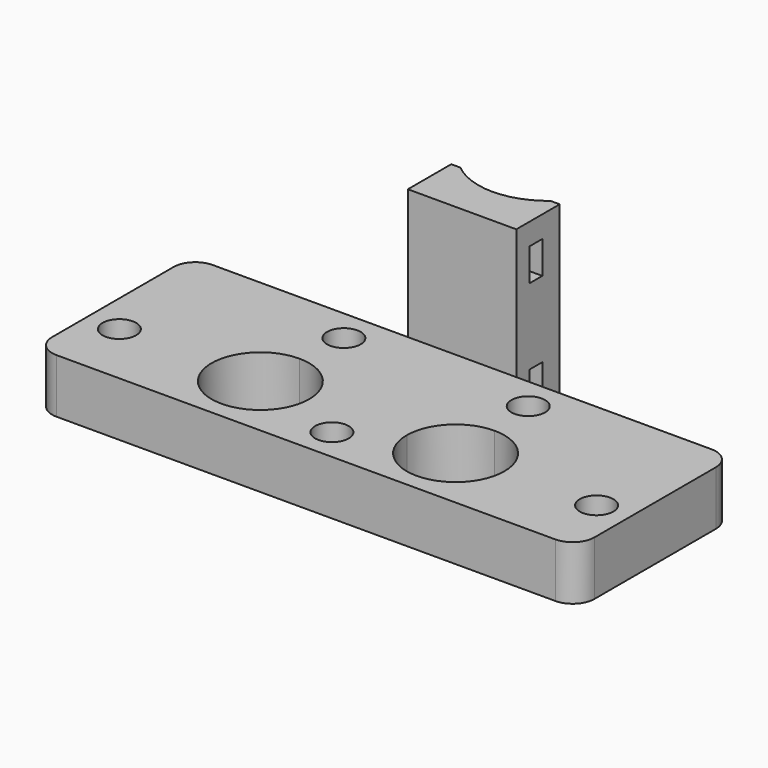
from build123d import *

# Parameters (mm, degrees)
F0_R          = 1.55
F1_DEPTH      = 5
F2_DEPTH      = 4
F3_DEPTH      = 17
F4_W          = 1.5
F4_H          = 3
F5_DEPTH      = 25
F6_W          = 1.52
F6_H          = 2
F7_DEPTH      = 11
F8_F1_R       = 2
F8_F2_R       = 2
F8_F3_R       = 2
F8_F4_R       = 2
F8_2_T1_DEPTH = 14


# Not quite as in the source:
# - a fillet or chamfer that OpenCascade refuses, or shapes differently, is made with other operations: its cross-section is extruded or revolved along the edge and cut away or added
# - a feature names something its author has since deleted; it is built from what else it names


with BuildPart() as f1:
    # F0 (on Top) → F1 (new body)
    with BuildSketch(Plane.XY):
        Polygon((-10, 0), (0, 0), (0, 10.5), (0, 18), (-10, 18), align=None)
        with Locations((-7, 6)):
            Circle(F0_R, mode=Mode.SUBTRACT)
        with BuildLine():
            Line((0, 10.5), (0, 0))
            Line((0, 0), (10.5, 0))
            Line((10.5, 0), (10.5, 6))
            ThreePointArc((10.5, 6), (2.8180194847, 2.8180194847), (6, 10.5))
            Line((6, 10.5), (0, 10.5))
        make_face()
        with BuildLine():
            Line((10.5, 6), (10.5, 0))
            Line((10.5, 0), (19.5, 0))
            Line((19.5, 0), (19.5, 6))
            ThreePointArc((19.5, 6), (20.8180194847, 9.1819805153), (24, 10.5))
            Line((24, 10.5), (6, 10.5))
            ThreePointArc((6, 10.5), (9.1819805153, 9.1819805153), (10.5, 6))
        make_face()
        with Locations((15, 3)):
            Circle(F0_R, mode=Mode.SUBTRACT)
        with BuildLine():
            Line((19.5, 6), (19.5, 0))
            Line((19.5, 0), (30, 0))
            Line((30, 0), (30, 10.5))
            Line((30, 10.5), (24, 10.5))
            ThreePointArc((24, 10.5), (27.1819805153, 9.1819805153), (28.5, 6))
            ThreePointArc((28.5, 6), (24, 1.5), (19.5, 6))
        make_face()
        Polygon((30, 10.5), (30, 0), (40, 0), (40, 18), (30, 18), align=None)
        with Locations((37, 6)):
            Circle(F0_R, mode=Mode.SUBTRACT)
        Polygon((0, 18), (0, 10.5), (6, 10.5), (24, 10.5), (30, 10.5), (30, 18), (20, 18), (10, 18), align=None)
        with Locations((6.5, 15)):
            Circle(F0_R, mode=Mode.SUBTRACT)
        with Locations((23.5, 15)):
            Circle(F0_R, mode=Mode.SUBTRACT)
    extrude(amount=F1_DEPTH)

    # F0 (on Top) → F3 (join)
    with BuildSketch(Plane.XY):
        with BuildLine():
            Line((10, 23), (10, 18))
            Line((10, 18), (20, 18))
            Line((20, 18), (20, 23))
            Line((20, 23), (19.1533119315, 23))
            ThreePointArc((19.1533119315, 23), (15, 21.5), (10.8466880685, 23))
            Line((10.8466880685, 23), (10, 23))
        make_face()
    extrude(amount=F3_DEPTH)

    # F4 (on face) → F5 (cut)
    with BuildSketch(Plane(origin=(10, 0, 0), x_dir=(0, -1, 0), z_dir=(-1, 0, 0))):
        with Locations((-20.25, 3.5)):
            Rectangle(F4_W, F4_H)
        with Locations((-20.25, 13.5)):
            Rectangle(F4_W, F4_H)
    extrude(amount=-F5_DEPTH, mode=Mode.SUBTRACT)

    # F8: fillet of radius 2 on 4 edges, made by hand

    # F8_f1
    f8_f1_edges = [f1.edges().sort_by_distance(p)[0] for p in [
        (40, 0, 2.5),
    ]]
    fillet(f8_f1_edges, radius=F8_F1_R)

    # F8_f2
    f8_f2_edges = [f1.edges().sort_by_distance(p)[0] for p in [
        (40, 18, 2.5),
    ]]
    fillet(f8_f2_edges, radius=F8_F2_R)

    # F8_f3
    f8_f3_edges = [f1.edges().sort_by_distance(p)[0] for p in [
        (-10, 0, 2.5),
    ]]
    fillet(f8_f3_edges, radius=F8_F3_R)

    # F8_f4
    f8_f4_edges = [f1.edges().sort_by_distance(p)[0] for p in [
        (-10, 18, 2.5),
    ]]
    fillet(f8_f4_edges, radius=F8_F4_R)


with BuildPart() as f2:
    # F0 (on Top) → F2 (new body)
    with BuildSketch(Plane.XY):
        Polygon((0, 18), (0, 10.5), (6, 10.5), (24, 10.5), (30, 10.5), (30, 18), (20, 18), (10, 18), align=None)
        with Locations((6.5, 15)):
            Circle(F0_R, mode=Mode.SUBTRACT)
        with Locations((23.5, 15)):
            Circle(F0_R, mode=Mode.SUBTRACT)
    extrude(amount=-F2_DEPTH)

    # F6 (on face) → F7 (cut)
    with BuildSketch(Plane(origin=(0, 18, 0), x_dir=(-1, 0, 0), z_dir=(0, 1, 0))):
        with Locations((-3.48, -2)):
            Rectangle(F6_W, F6_H)
        with Locations((-5.4, -2)):
            Rectangle(F6_W, F6_H)
        with Locations((-7.32, -2)):
            Rectangle(F6_W, F6_H)
        with Locations((-9.24, -2)):
            Rectangle(F6_W, F6_H)
        with Locations((-11.16, -2)):
            Rectangle(F6_W, F6_H)
        with Locations((-13.08, -2)):
            Rectangle(F6_W, F6_H)
        with Locations((-15, -2)):
            Rectangle(F6_W, F6_H)
        with Locations((-16.92, -2)):
            Rectangle(F6_W, F6_H)
        with Locations((-18.84, -2)):
            Rectangle(F6_W, F6_H)
        with Locations((-20.76, -2)):
            Rectangle(F6_W, F6_H)
        with Locations((-22.68, -2)):
            Rectangle(F6_W, F6_H)
        with Locations((-24.6, -2)):
            Rectangle(F6_W, F6_H)
        with Locations((-26.52, -2)):
            Rectangle(F6_W, F6_H)
        with Locations((-28.44, -2)):
            Rectangle(F6_W, F6_H)
        with Locations((-1.56, -2)):
            Rectangle(F6_W, F6_H)
    extrude(amount=-F7_DEPTH, mode=Mode.SUBTRACT)

    # F8#2: fillet of radius 2 on 4 edges, made by hand

    # F8_2_s2 → F8_2_t1 (cut)
    with BuildSketch(Plane.XY.offset(-9)):
        with BuildLine():
            ThreePointArc((0, 16), (0.5857864376, 17.4142135624), (2, 18))
            Line((2, 18), (0, 18))
            Line((0, 18), (0, 16))
        make_face()
        with BuildLine():
            ThreePointArc((28, 18), (29.4142135624, 17.4142135624), (30, 16))
            Line((30, 16), (30, 18))
            Line((30, 18), (28, 18))
        make_face()
        with BuildLine():
            ThreePointArc((28, 10.5), (29.4142135624, 11.0857864376), (30, 12.5))
            Line((30, 12.5), (30, 10.5))
            Line((30, 10.5), (28, 10.5))
        make_face()
        with BuildLine():
            ThreePointArc((0, 12.5), (0.5857864376, 11.0857864376), (2, 10.5))
            Line((2, 10.5), (0, 10.5))
            Line((0, 10.5), (0, 12.5))
        make_face()
    extrude(amount=F8_2_T1_DEPTH, mode=Mode.SUBTRACT)


solid = Compound([f1.part, f2.part])
